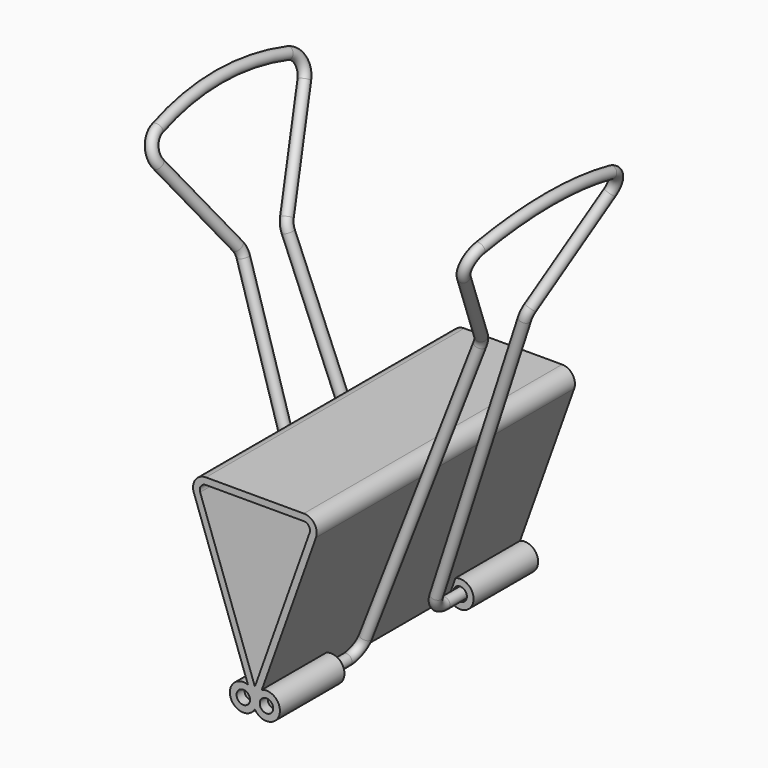
from build123d import *

# Parameters (mm, degrees)
F1_DEPTH         = 9.525
F2_R             = 0.762
F3_T             = -0.396875
F5_DEPTH         = 19.051
F7_DEPTH         = 4.7625
F7_COPIES2_COUNT = 2
F8_R             = 0.396875
F9_DEPTH         = 19.051
F14_R            = 0.3175


# Not quite as in the source:
# - a pattern or mirror of a feature is missing from the dataset's text; its kind, count and spacing are read off the source's solid


with BuildPart() as f1:
    # F0 (on Front) → F1 (new body, symmetric)
    with BuildSketch(Plane.XZ):
        Polygon((-3.96875, 11.1125), (0, 0), (3.96875, 11.1125), align=None)
    extrude(amount=F1_DEPTH, both=True)

    # F2
    f2_edges = [f1.edges().sort_by_distance(p)[0] for p in [
        (3.96875, 0, 11.1125),
        (-3.96875, 0, 11.1125),
    ]]
    fillet(f2_edges, radius=F2_R)

    # F3
    f3_openings = [f1.faces().sort_by_distance(p)[0] for p in [
        (0, -9.525, 7.365674),
    ]]
    offset(amount=F3_T, openings=f3_openings)

    # F4 (on face) → F5 (cut, through all)
    with BuildSketch(Plane(origin=(0, 9.525, 0), x_dir=(-1, 0, 0), z_dir=(0, 1, 0))):
        with BuildLine():
            ThreePointArc((3.2313217737, 10.227695173), (3.1859271147, 10.5608296855), (2.8874682582, 10.715625))
            Line((2.8874682582, 10.715625), (-2.8874682582, 10.715625))
            ThreePointArc((-2.8874682582, 10.715625), (-3.1859271147, 10.5608296855), (-3.2313217737, 10.227695173))
            Line((-3.2313217737, 10.227695173), (0, 1.1799942068))
            Line((0, 1.1799942068), (3.2313217737, 10.227695173))
        make_face()
    extrude(amount=-F5_DEPTH, mode=Mode.SUBTRACT)

    # F6 (on face) → F7 (join)
    with BuildSketch(Plane.XZ.offset(9.525)):
        with BuildLine():
            Line((0.4102615116, 1.1487322325), (0, 0))
            ThreePointArc((0, 0), (1.4310432892, 0.1365402115), (0.4102615116, 1.1487322325))
        make_face()
    f7 = extrude(amount=-F7_DEPTH)

    # F7_copies: F7 across plane
    add(f7.mirror(Plane(origin=(0, 0, 0), x_dir=(0, 0, -1), z_dir=(-1, 0, 0))))

    # F7_copies1: F7 across plane
    add(f7.mirror(Plane.ZX))

    # F7_copies2: F7 ×2 about axis
    f7_copies2_axis = Axis((0, 0, 0), (0, 0, 1))
    for i in range(1, F7_COPIES2_COUNT):
        add(f7.rotate(f7_copies2_axis, i * 360 / F7_COPIES2_COUNT))

    # F8 (on face) → F9 (cut, through all)
    with BuildSketch(Plane.XZ.offset(9.525)):
        with Locations((0.6835356469, 0.4035072266)):
            Circle(F8_R)
    f9 = extrude(amount=-F9_DEPTH, mode=Mode.SUBTRACT)

    # F9_copies: F9 across plane
    add(f9.mirror(Plane(origin=(0, 0, 0), x_dir=(0, 0, -1), z_dir=(-1, 0, 0))), mode=Mode.SUBTRACT)


with BuildPart() as f15:
    # F15: sweep along a path in F12
    with BuildLine(Plane(origin=(0.4784048911, 0, -0.1708588897), x_dir=(0, 1, 0), z_dir=(0.9417419116, 0, -0.336336397))) as f15_path:
        Line((-9.0260086581, 0.6098975836), (-3.6195, 0.6098975836))
        ThreePointArc((-3.6195, 0.6098975836), (-2.9205872332, 0.8884852537), (-2.6049588744, 1.5714705278))
        Line((-2.6049588744, 1.5714705278), (-1.6524588744, 19.326434617))
        ThreePointArc((-1.6524588744, 19.326434617), (-1.6861909522, 19.6459458327), (-1.8180036213, 19.9389487171))
        Line((-1.8180036213, 19.9389487171), (-5.3892463787, 25.3717431168))
        ThreePointArc((-5.3892463787, 25.3717431168), (-5.4939189383, 26.2802178837), (-4.825976101, 26.9048258509))
        ThreePointArc((-4.825976101, 26.9048258509), (0, 27.5973975836), (4.825976101, 26.9048258509))
        ThreePointArc((4.825976101, 26.9048258509), (5.4939189383, 26.2802178837), (5.3892463787, 25.3717431168))
        Line((5.3892463787, 25.3717431168), (1.8180036213, 19.9389487171))
        ThreePointArc((1.8180036213, 19.9389487171), (1.6861909522, 19.6459458327), (1.6524588744, 19.326434617))
        Line((1.6524588744, 19.326434617), (2.6049588744, 1.5714705278))
        ThreePointArc((2.6049588744, 1.5714705278), (2.9205872332, 0.8884852537), (3.6195, 0.6098975836))
        Line((3.6195, 0.6098975836), (9.0260086581, 0.6098975836))
    # F14 (on face) → F15 (sweep)
    with BuildSketch(Plane.XZ.offset(9.0260086581)):
        with Locations((0.6835356469, 0.4035072266)):
            Circle(F14_R)
    sweep(path=f15_path.line)


with BuildPart() as f16_1:
    # F16: instance of F15
    add(f15.part.mirror(Plane.YZ))


solid = Compound([f1.part, f15.part, f16_1.part])
